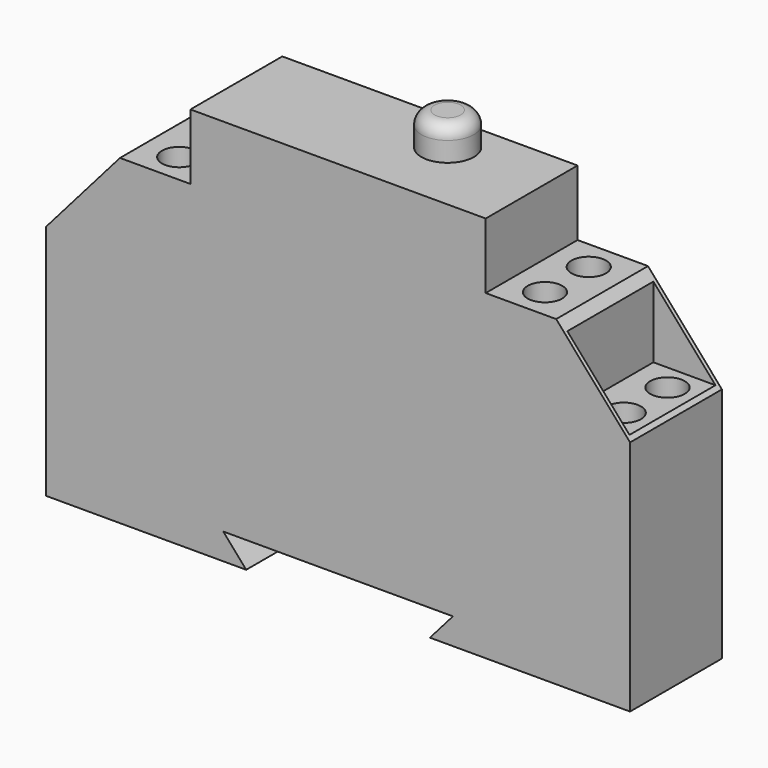
from build123d import *

# Parameters (mm, degrees)
F1_DEPTH = 8.75
F2_W     = 16.3845960051
F2_H     = 5.8396488756
F3_DEPTH = 10
F4_W     = 16.0876363516
F4_H     = 5.6553587645
F5_DEPTH = 10
F6_R     = 2.6324784905
F7_DEPTH = 25
F8_R     = 4
F9_DEPTH = 5
F10_R    = 2


# Not quite as in the source:
# - a feature names something its author has since deleted; it is built from what else it names


with BuildPart() as f1:
    # F0 (on Front) → F1 (new body, symmetric)
    with BuildSketch(Plane.XZ):
        Polygon((22.5, 19.5), (22.5, 29.5), (-22.5, 29.5), (-22.5, 19.5), (-33.2391485572, 19.5), (-44.5, 6.6135488451), (-44.5, -29.5), (-14, -29.5), (-17.5, -25.5), (17.5, -25.5), (14, -29.5), (44.5, -29.5), (44.5, 6.6135488451), (33.2391485572, 19.5), align=None)
    extrude(amount=F1_DEPTH, both=True)

    # F2 (on face) → F3 (cut)
    with BuildSketch(Plane.YZ.offset(44.5)):
        with Locations((0, 15.9833732828)):
            Rectangle(F2_W, F2_H)
        with Locations((0, 10.1437244073)):
            Rectangle(F2_W, F2_H)
    extrude(amount=-F3_DEPTH, mode=Mode.SUBTRACT)

    # F4 (on face) → F5 (cut)
    with BuildSketch(Plane(origin=(-44.5, 0, 0), x_dir=(0, -1, 0), z_dir=(-1, 0, 0))):
        with Locations((0, 15.8912282273)):
            Rectangle(F4_W, F4_H)
        with Locations((0, 10.2358694628)):
            Rectangle(F4_W, F4_H)
    extrude(amount=-F5_DEPTH, mode=Mode.SUBTRACT)

    # F6 (on face) → F7 (cut)
    with BuildSketch(Plane.XY.offset(19.5)):
        with BuildLine():
            ThreePointArc((-25.2370957881, -4.1691302322), (-26.0081308866, -2.3076868402), (-27.8695742786, -1.5366517417))
            Line((-27.8695742786, -1.5366517417), (-27.8695742786, -6.8016087227))
            ThreePointArc((-27.8695742786, -6.8016087227), (-26.0081308866, -6.0305736241), (-25.2370957881, -4.1691302322))
        make_face()
        with BuildLine():
            Line((-27.8695742786, -6.8016087227), (-27.8695742786, -1.5366517417))
            ThreePointArc((-27.8695742786, -1.5366517417), (-30.5020527691, -4.1691302322), (-27.8695742786, -6.8016087227))
        make_face()
        with BuildLine():
            Line((-27.8695742786, 1.5366517417), (-27.8695742786, 6.8016087227))
            ThreePointArc((-27.8695742786, 6.8016087227), (-30.5020527691, 4.1691302322), (-27.8695742786, 1.5366517417))
        make_face()
        with BuildLine():
            ThreePointArc((-25.2370957881, 4.1691302322), (-26.0081308866, 6.0305736241), (-27.8695742786, 6.8016087227))
            Line((-27.8695742786, 6.8016087227), (-27.8695742786, 1.5366517417))
            ThreePointArc((-27.8695742786, 1.5366517417), (-26.0081308866, 2.3076868402), (-25.2370957881, 4.1691302322))
        make_face()
        with Locations((-39.8695742786, 4.1691302322)):
            Circle(F6_R)
        with Locations((-39.8695742786, -4.1691302322)):
            Circle(F6_R)
        with Locations((27.8695742786, 4.1691302322)):
            Circle(F6_R)
        with Locations((27.8695742786, -4.1691302322)):
            Circle(F6_R)
        with Locations((39.8695742786, 4.1691302322)):
            Circle(F6_R)
        with Locations((39.8695742786, -4.1691302322)):
            Circle(F6_R)
    extrude(amount=-F7_DEPTH, mode=Mode.SUBTRACT)

    # F8 (on face) → F9 (join)
    with BuildSketch(Plane.XY.offset(29.5)):
        with Locations((7.5, 2.75)):
            Circle(F8_R)
    extrude(amount=F9_DEPTH)

    # F10
    f10_edges = [f1.edges().sort_by_distance(p)[0] for p in [
        (3.5, 2.75, 34.5),
    ]]
    fillet(f10_edges, radius=F10_R)


solid = f1.part
